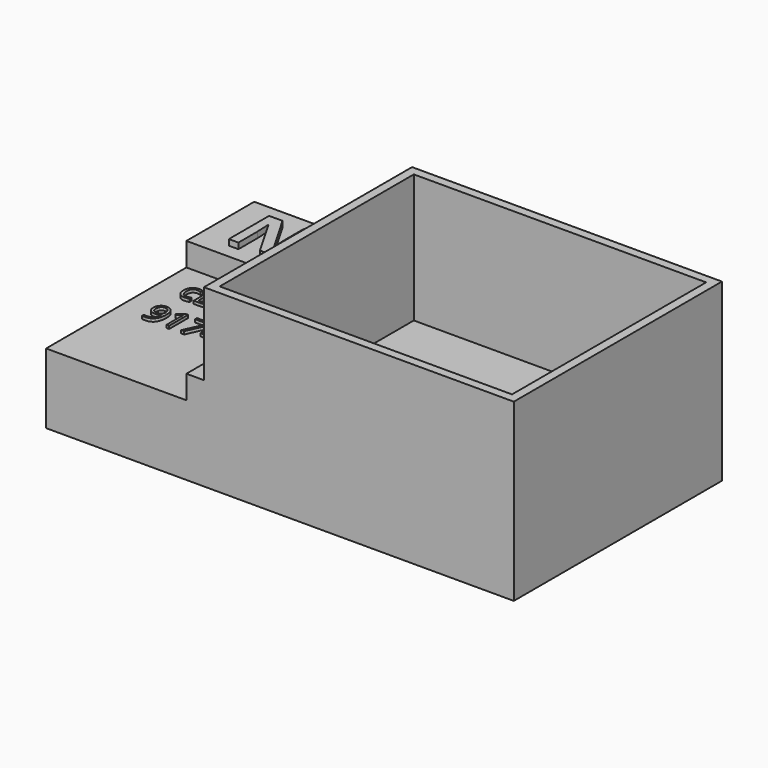
from build123d import *

# Parameters (mm, degrees)
F0_W          = 160
F0_H          = 89
F1_DEPTH      = 60
F2_W          = 54
F2_H          = 28
F3_DEPTH      = 89.001
F4_W          = 48
F4_H          = 8
F5_DEPTH      = 60
F7_DEPTH      = 44
F8_TEXT_SIZE  = 24.0887308286
F9_DEPTH      = 2
F10_TEXT_SIZE = 11.3291821132
F11_DEPTH     = 1


# Not quite as in the source:
# - Text() gives the source's letters only with a copy of the font that has no kerning and outlines rounded to 1/6400 em; it was checked with that copy


with BuildPart() as f1:
    # F0 (on Top) → F1 (new body)
    with BuildSketch(Plane.XY):
        with Locations((80, 44.5)):
            Rectangle(F0_W, F0_H)
    extrude(amount=F1_DEPTH)

    # F2 (on face) → F3 (cut, through all)
    with BuildSketch(Plane.XZ):
        with Locations((27, 46)):
            Rectangle(F2_W, F2_H)
    extrude(amount=-F3_DEPTH, mode=Mode.SUBTRACT)

    # F4 (on face) → F5 (cut)
    with BuildSketch(Plane.XZ):
        with Locations((24, 28)):
            Rectangle(F4_W, F4_H)
    extrude(amount=-F5_DEPTH, mode=Mode.SUBTRACT)

    # F6 (on face) → F7 (cut)
    with BuildSketch(Plane.XY.offset(60)):
        Polygon((57, 86), (57, 44.5), (57, 3), (107, 3), (157, 3), (157, 44.5), (157, 86), (107, 86), align=None)
    extrude(amount=-F7_DEPTH, mode=Mode.SUBTRACT)

    # F8 (on face) → F9 (join)
    with BuildSketch(Plane.XY.offset(32)):
        with Locations((8.4316506982, 64.9161860347)):
            Text('NI', F8_TEXT_SIZE, font='Open Sans', font_style=FontStyle.BOLD, text_align=(TextAlign.LEFT, TextAlign.BOTTOM))
    extrude(amount=F9_DEPTH)

    # F10 (on face) → F11 (join)
    with BuildSketch(Plane.XY.offset(24)):
        with Locations((8.2246572711, 44.7279326618)):
            Text('cDAQ', F10_TEXT_SIZE, font='Open Sans', text_align=(TextAlign.LEFT, TextAlign.BOTTOM))
        with Locations((8.2246572711, 29.3202449878)):
            Text('9174', F10_TEXT_SIZE, font='Open Sans', text_align=(TextAlign.LEFT, TextAlign.BOTTOM))
    extrude(amount=F11_DEPTH)


solid = f1.part
